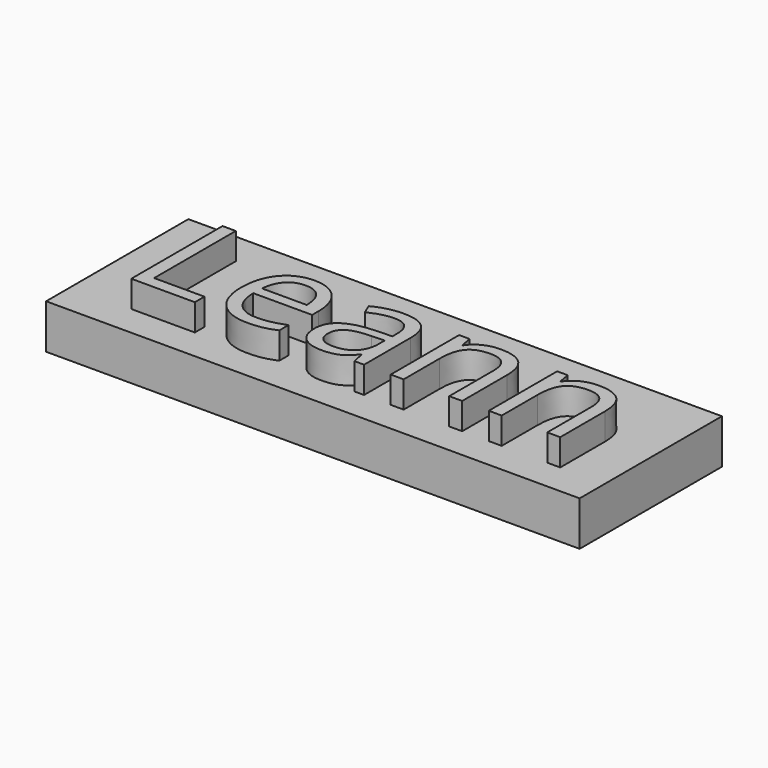
from build123d import *

# Parameters (mm, degrees)
F0_W         = 60
F0_H         = 20
F1_DEPTH     = 5
F2_TEXT_SIZE = 17.9644080166
F3_DEPTH     = 3


# Not quite as in the source:
# - Text() gives the source's letters only with a copy of the font that has no kerning and outlines rounded to 1/6400 em; it was checked with that copy


with BuildPart() as f1:
    # F0 (on Top) → F1 (new body)
    with BuildSketch(Plane.XY):
        Rectangle(F0_W, F0_H)
    extrude(amount=F1_DEPTH)

    # F2 (on face) → F3 (join)
    with BuildSketch(Plane.XY.offset(5)):
        with Locations((-25, -6.4782051242)):
            Text('Leann', F2_TEXT_SIZE, font='Open Sans', text_align=(TextAlign.LEFT, TextAlign.BOTTOM))
    extrude(amount=F3_DEPTH)


solid = f1.part
